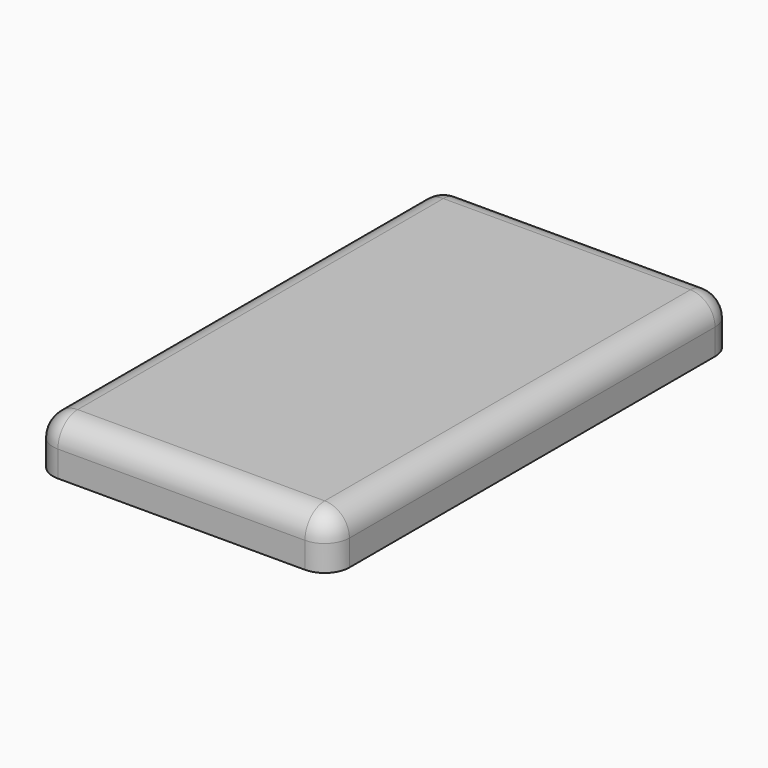
from build123d import *

# Parameters (mm, degrees)
F0_R     = 17.78
F0_W     = 50.8
F0_H     = 38.1
F0_R_2   = 7.62
F1_DEPTH = 10.414
F2_R     = 5.08


with BuildPart() as f1:
    # F0 (on Top) → F1 (new body)
    with BuildSketch(Plane.XY):
        with BuildLine():
            Line((-10.817469722, 14.821465837), (-61.617469722, 14.821465837))
            ThreePointArc((-61.617469722, 14.821465837), (-65.2095721705, 13.3335682854), (-66.697469722, 9.741465837))
            Line((-66.697469722, 9.741465837), (-66.697469722, -84.238534163))
            ThreePointArc((-66.697469722, -84.238534163), (-65.2095721705, -87.8306366114), (-61.617469722, -89.318534163))
            Line((-61.617469722, -89.318534163), (-10.817469722, -89.318534163))
            ThreePointArc((-10.817469722, -89.318534163), (-7.2253672736, -87.8306366114), (-5.737469722, -84.238534163))
            Line((-5.737469722, -84.238534163), (-5.737469722, 9.741465837))
            ThreePointArc((-5.737469722, 9.741465837), (-7.2253672736, 13.3335682854), (-10.817469722, 14.821465837))
        make_face()
        with Locations((-36.217469722, -58.838534163)):
            Circle(F0_R, mode=Mode.SUBTRACT)
        with Locations((-36.217469722, -10.578534163)):
            Rectangle(F0_W, F0_H, mode=Mode.SUBTRACT)
        with Locations((-36.217469722, -10.578534163)):
            Rectangle(F0_W, F0_H)
        with Locations((-36.217469722, -58.838534163)):
            Circle(F0_R)
        with Locations((-36.217469722, -58.838534163)):
            Circle(F0_R_2, mode=Mode.SUBTRACT)
        with Locations((-36.217469722, -58.838534163)):
            Circle(F0_R_2)
    extrude(amount=F1_DEPTH)

    # F2
    f2_edges = [f1.edges().sort_by_distance(p)[0] for p in [
        (-36.21747, -89.318534, 10.414),
        (-36.21747, 14.821466, 10.414),
    ]]
    fillet(f2_edges, radius=F2_R)


solid = f1.part
